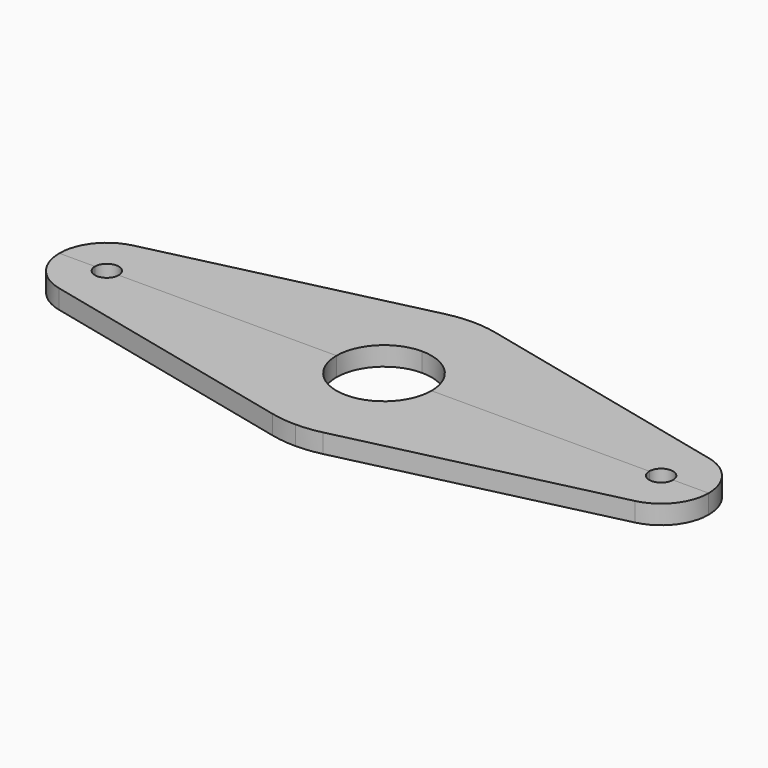
from build123d import *
from build123d import SkipClean  # not in build123d's __all__

# Parameters (mm, degrees)
F1_DEPTH = 1.2


with BuildPart() as f1:
    # F0 (on Top) → F1 (new body)
    with BuildSketch(Plane.XY):
        with BuildLine():
            ThreePointArc((0, -7), (0.8053477185, -6.953518178), (1.6, -6.814690015))
            Line((1.6, -6.814690015), (18.1857142857, -2.920581435))
            ThreePointArc((18.1857142857, -2.920581435), (19.8512914385, -1.8631770102), (20.5, 0))
            Line((20.5, 0), (18.25, 0))
            ThreePointArc((18.25, 0), (17.5, -0.75), (16.75, 0))
            Line((16.75, 0), (3, 0))
            ThreePointArc((3, 0), (2.1213203436, -2.1213203436), (0, -3))
            Line((0, -3), (0, -7))
        make_face()
    extrude(amount=F1_DEPTH)

    # F2: F1 across plane


with BuildPart() as f1_1:
    add(f1.part, clean=False)
    add(f1.part.mirror(Plane.YZ), clean=False)

    # F3: F1 across plane


with BuildPart() as f1_2:
    add(f1_1.part, clean=False)
    with SkipClean():  # cleaning this boolean's faces spoils the solid; the shape is the same uncleaned
        add(f1_1.part.mirror(Plane.XZ), clean=False)


solid = f1_2.part
